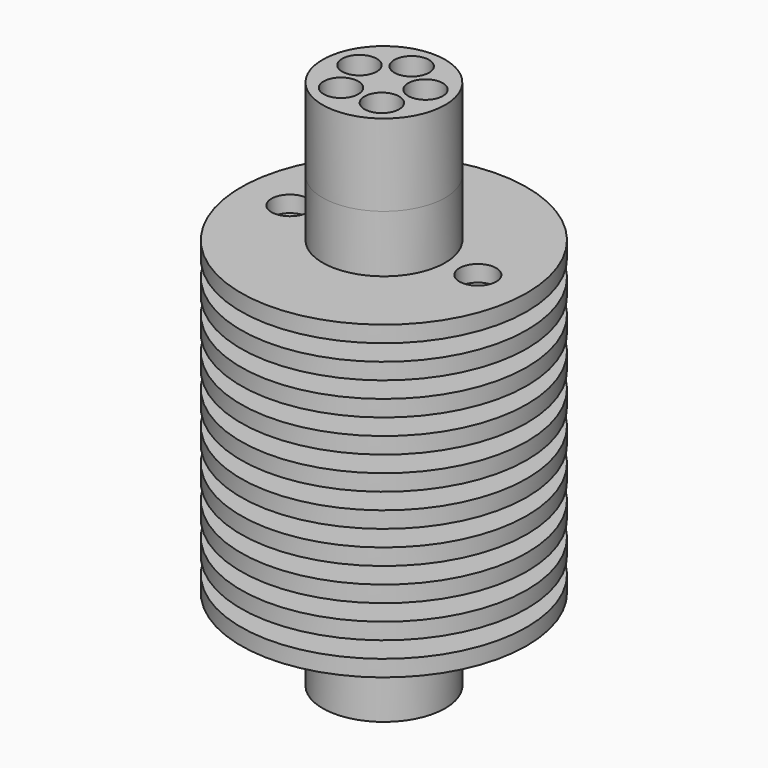
from build123d import *

# Parameters (mm, degrees)
F0_R     = 7.5
F0_R_2   = 2
F1_DEPTH = 50
F2_W     = 10
F2_H     = 2
F4_DEPTH = 5
F6_D     = 2
F7_D     = 4.5
F7_DEPTH = 22
F7_TIP   = 1.3519363928
F8_DEPTH = 10
F10_D    = 4.25


# Not quite as in the source:
# - a feature names something its author has since deleted; it is built from what else it names


with BuildPart() as f1:
    # F0 (on Top) → F1 (new body)
    with BuildSketch(Plane.XY):
        Circle(F0_R)
        with Locations((-2.4980873222, -3.4383222261)):
            Circle(F0_R_2, mode=Mode.SUBTRACT)
        with Locations((2.4980873222, -3.4383222261)):
            Circle(F0_R_2, mode=Mode.SUBTRACT)
        with Locations((-4.0419901943, 1.3133222261)):
            Circle(F0_R_2, mode=Mode.SUBTRACT)
        with Locations((4.0419901943, 1.3133222261)):
            Circle(F0_R_2, mode=Mode.SUBTRACT)
        with BuildLine():
            ThreePointArc((0, 2.25), (-1.4142135624, 5.6642135624), (2, 4.25))
            ThreePointArc((2, 4.25), (1.4142135624, 2.8357864376), (0, 2.25))
        make_face(mode=Mode.SUBTRACT)
    extrude(amount=F1_DEPTH)

    # F2 (on Front) → F3 (revolve)
    with BuildSketch(Plane.XZ):
        with Locations((12.5, 6)):
            Rectangle(F2_W, F2_H)
        with Locations((12.5, 10)):
            Rectangle(F2_W, F2_H)
        with Locations((12.5, 14)):
            Rectangle(F2_W, F2_H)
        with Locations((12.5, 18)):
            Rectangle(F2_W, F2_H)
        with Locations((12.5, 22)):
            Rectangle(F2_W, F2_H)
        with Locations((12.5, 26)):
            Rectangle(F2_W, F2_H)
        with Locations((12.5, 30)):
            Rectangle(F2_W, F2_H)
        with Locations((12.5, 34)):
            Rectangle(F2_W, F2_H)
        with Locations((12.5, 38)):
            Rectangle(F2_W, F2_H)
        with Locations((12.5, 42)):
            Rectangle(F2_W, F2_H)
    revolve(axis=Axis((0, 0, 30.4011311382), (0, 0, 1)))

    # F4 (add): a face of the model
    f4_faces = [f1.faces().sort_by_distance(p)[0] for p in [
        (0, 0, 0),
    ]]
    extrude(f4_faces, amount=F4_DEPTH)

    # F6 (through all)
    with Locations(Plane.XY.offset(43)):
        with Locations((-11.5, 0), (11.5, 0)):
            Hole(F6_D / 2)

    # F7
    with Locations(Plane.XY.offset(43)):
        with Locations((-11.5, 0), (11.5, 0)):
            Hole(F7_D / 2, depth=F7_DEPTH)
            with Locations((0, 0, -(F7_DEPTH + F7_TIP / 2))):  # 118° drill point
                Cone(0, F7_D / 2, F7_TIP, mode=Mode.SUBTRACT)


with BuildPart() as f8:
    # F8 (new): a face of the model
    f8_faces = [f1.part.faces().sort_by_distance(p)[0] for p in [
        (0, 0, 50),
    ]]
    extrude(f8_faces, amount=F8_DEPTH)

    # F10 (through all)
    with Locations(Plane.XY.offset(60)):
        with Locations((0, 4.25), (4.0419901943, 1.3133222261), (2.4980873222, -3.4383222261), (-2.4980873222, -3.4383222261), (-4.0419901943, 1.3133222261)):
            Hole(F10_D / 2)


solid = Compound([f1.part, f8.part])
